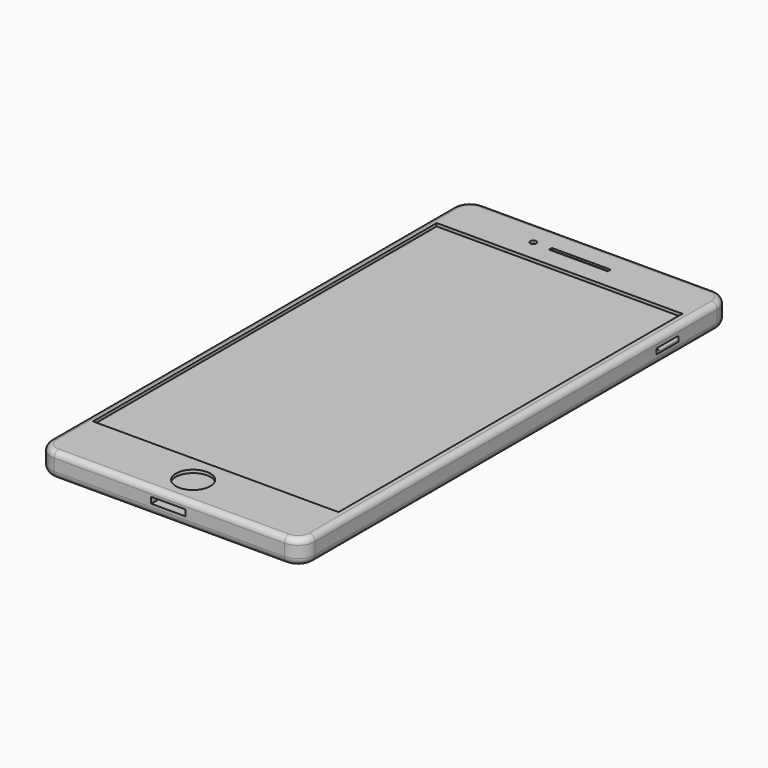
from build123d import *

# Parameters (mm, degrees)
F0_W         = 77.9
F0_H         = 158.2
F1_DEPTH     = 7.3
F2_R         = 5
F3_R         = 1.6899494937
F4_R         = 2.1727922061
F5_W         = 72.4303945899
F5_H         = 126.6588754952
F6_DEPTH     = 0.9
F7_R         = 5.0823894813
F8_DEPTH     = 0.9
F9_W         = 17.3039510846
F9_H         = 1.0814964771
F10_DEPTH    = 0.6
F11_R        = 0.8966339166
F12_DEPTH    = 0.8
F13_W        = 17.3039520159
F13_H        = 4.6321238935
F14_DEPTH    = 1.7
F15_R        = 0.7242640687
F16_R        = 1.0910584654
F17_DEPTH    = 1.2
F18_R        = 1.1204591048
F18_R_2      = 0.2597799208
F19_DEPTH    = 0.5
F20_R        = 0.5652467708
F21_DEPTH    = 1.3
F22_R        = 1.5140930758
F23_DEPTH    = 0.6
F24_W        = 10.0857308134
F24_H        = 1.8002798315
F25_DEPTH    = 8.7
F26_W        = 7.992297411
F26_H        = 1.5090261586
F27_DEPTH    = 0.5
F28_T1_DEPTH = 5.0389206483
F28_T3_DEPTH = 11.5221919007
F29_R        = 1.0914541248
F30_DEPTH    = 0.9
F31_R        = 1.1331057204
F32_DEPTH    = 0.8
F33_W        = 73.5544155877
F33_H        = 1.0814964771
F34_DEPTH    = 0.4


# Not quite as in the source:
# - a fillet or chamfer that OpenCascade refuses, or shapes differently, is made with other operations: its cross-section is extruded or revolved along the edge and cut away or added


with BuildPart() as f1:
    # F0 (on Top) → F1 (new body)
    with BuildSketch(Plane.XY):
        with Locations((-9.3765874773, -13.58352229)):
            Rectangle(F0_W, F0_H)
    extrude(amount=F1_DEPTH)

    # F2
    f2_edges = [f1.edges().sort_by_distance(p)[0] for p in [
        (-48.326587, -92.683522, 3.65),
        (29.573413, -92.683522, 3.65),
        (29.573413, 65.516478, 3.65),
        (-48.326587, 65.516478, 3.65),
    ]]
    fillet(f2_edges, radius=F2_R)

    # F3
    f3_edges = [f1.edges().sort_by_distance(p)[0] for p in [
        (-48.326587, -13.583522, 7.3),
        (-9.376587, 65.516478, 7.3),
        (28.108946, 64.052012, 7.3),
        (-46.862121, 64.052012, 7.3),
        (29.573413, -13.583522, 7.3),
        (28.108946, -91.219056, 7.3),
        (-46.862121, -91.219056, 7.3),
        (-9.376587, -92.683522, 7.3),
    ]]
    fillet(f3_edges, radius=F3_R)

    # F4
    f4_edges = [f1.edges().sort_by_distance(p)[0] for p in [
        (-48.326587, -13.583522, 0),
        (-9.376587, 65.516478, 0),
        (28.108946, 64.052012, 0),
        (-46.862121, 64.052012, 0),
        (29.573413, -13.583522, 0),
        (28.108946, -91.219056, 0),
        (-46.862121, -91.219056, 0),
        (-9.376587, -92.683522, 0),
    ]]
    fillet(f4_edges, radius=F4_R)

    # F5 (on face) → F6 (cut)
    with BuildSketch(Plane.XY.offset(7.3)):
        with Locations((-9.5828361809, -11.9932051748)):
            Rectangle(F5_W, F5_H)
    extrude(amount=-F6_DEPTH, mode=Mode.SUBTRACT)

    # F7 (on face) → F8 (cut)
    with BuildSketch(Plane.XY.offset(7.3)):
        with Locations((-9.5828361809, -83.671361208)):
            Circle(F7_R)
    extrude(amount=-F8_DEPTH, mode=Mode.SUBTRACT)

    # F9 (on face) → F10 (cut)
    with BuildSketch(Plane.XY.offset(7.3)):
        with Locations((-8.6519755423, 57.6703026891)):
            Rectangle(F9_W, F9_H)
    extrude(amount=-F10_DEPTH, mode=Mode.SUBTRACT)

    # F11 (on face) → F12 (cut)
    with BuildSketch(Plane.XY.offset(7.3)):
        with Locations((-22.4402733147, 57.7334612608)):
            Circle(F11_R)
    extrude(amount=-F12_DEPTH, mode=Mode.SUBTRACT)

    # F13 (on face) → F14 (join)
    with BuildSketch(Plane(origin=(0, 0, 0), x_dir=(1, 0, 0), z_dir=(0, 0, -1))):
        with Locations((11.9729838334, -58.2004157633)):
            Rectangle(F13_W, F13_H)
    extrude(amount=F14_DEPTH)

    # F15
    f15_edges = [f1.edges().sort_by_distance(p)[0] for p in [
        (11.972984, 60.516478, -1.7),
        (11.972984, 55.884354, -1.7),
        (20.62496, 58.200416, -1.7),
        (3.321008, 58.200416, -1.7),
    ]]
    fillet(f15_edges, radius=F15_R)

    # F16 (on face) → F17 (cut)
    with BuildSketch(Plane(origin=(0, 0, -1.7), x_dir=(1, 0, 0), z_dir=(0, 0, -1))):
        with Locations((17.652342096, -58.0027028918)):
            Circle(F16_R)
    extrude(amount=-F17_DEPTH, mode=Mode.SUBTRACT)

    # F18 (on face) → F19 (cut)
    with BuildSketch(Plane(origin=(0, 0, -1.7), x_dir=(1, 0, 0), z_dir=(0, 0, -1))):
        with Locations((13.1328506395, -57.9593703151)):
            Circle(F18_R)
        with Locations((13.1328506395, -57.9593703151)):
            Circle(F18_R_2, mode=Mode.SUBTRACT)
    extrude(amount=-F19_DEPTH, mode=Mode.SUBTRACT)

    # F20 (on face) → F21 (cut)
    with BuildSketch(Plane(origin=(0, 0, 0), x_dir=(1, 0, 0), z_dir=(0, 0, -1))):
        with Locations((0, -57.881783694)):
            Circle(F20_R)
    extrude(amount=-F21_DEPTH, mode=Mode.SUBTRACT)

    # F22 (on face) → F23 (cut)
    with BuildSketch(Plane(origin=(0, 0, 0), x_dir=(1, 0, 0), z_dir=(0, 0, -1))):
        with Locations((-3.8621318527, -57.8266605735)):
            Circle(F22_R)
    extrude(amount=-F23_DEPTH, mode=Mode.SUBTRACT)

    # F24 (on face) → F25 (cut)
    with BuildSketch(Plane.XZ.offset(92.68352229)):
        with Locations((-9.6801561303, 3.9914349327)):
            Rectangle(F24_W, F24_H)
    extrude(amount=-F25_DEPTH, mode=Mode.SUBTRACT)

    # F26 (on face) → F27 (join)
    with BuildSketch(Plane.YZ.offset(29.5734125227)):
        with Locations((42.0706942677, 3.8539019879)):
            Rectangle(F26_W, F26_H)
    extrude(amount=F27_DEPTH)

    # F28: fillet of radius 0.7484062043 on 4 edges, made by hand

    # F28_s2 → F28_t1 (cut)
    with BuildSketch(Plane.XY.offset(1.3344416637)):
        with BuildLine():
            ThreePointArc((29.5734125227, 46.0668429732), (29.9357520066, 45.7934164433), (30.0734125227, 45.3608640753))
            Line((30.0734125227, 45.3608640753), (30.0734125227, 46.0668429732))
            Line((30.0734125227, 46.0668429732), (29.5734125227, 46.0668429732))
        make_face()
        with BuildLine():
            ThreePointArc((29.5734125227, 38.0745455623), (29.9357520066, 38.3479720922), (30.0734125227, 38.7805244602))
            Line((30.0734125227, 38.7805244602), (30.0734125227, 38.0745455623))
            Line((30.0734125227, 38.0745455623), (29.5734125227, 38.0745455623))
        make_face()
    extrude(amount=F28_T1_DEPTH, mode=Mode.SUBTRACT)

    # F28_s4 → F28_t3 (cut)
    with BuildSketch(Plane.XZ.offset(-47.8317902181)):
        with BuildLine():
            ThreePointArc((29.5734125227, 4.6084150672), (29.9357520066, 4.3349885373), (30.0734125227, 3.9024361693))
            Line((30.0734125227, 3.9024361693), (30.0734125227, 4.6084150672))
            Line((30.0734125227, 4.6084150672), (29.5734125227, 4.6084150672))
        make_face()
        with BuildLine():
            ThreePointArc((29.5734125227, 3.0993889086), (29.9357520066, 3.3728154385), (30.0734125227, 3.8053678065))
            Line((30.0734125227, 3.8053678065), (30.0734125227, 3.0993889086))
            Line((30.0734125227, 3.0993889086), (29.5734125227, 3.0993889086))
        make_face()
    extrude(amount=F28_T3_DEPTH, mode=Mode.SUBTRACT)

    # F29 (on face) → F30 (join)
    with BuildSketch(Plane(origin=(-48.3265874773, 0, 0), x_dir=(0, -1, 0), z_dir=(-1, 0, 0))):
        with Locations((-41.7392961681, 4.070978146)):
            Circle(F29_R)
    extrude(amount=F30_DEPTH)

    # F31 (on face) → F32 (join)
    with BuildSketch(Plane(origin=(-48.3265874773, 0, 0), x_dir=(0, -1, 0), z_dir=(-1, 0, 0))):
        with Locations((-36.7904044688, 4.1209622286)):
            Circle(F31_R)
    extrude(amount=F32_DEPTH)

    # F33 (on face) → F34 (cut)
    with BuildSketch(Plane(origin=(0, 0, 0), x_dir=(1, 0, 0), z_dir=(0, 0, -1))):
        with Locations((-9.3765874773, 75.3538236022)):
            Rectangle(F33_W, F33_H)
    extrude(amount=-F34_DEPTH, mode=Mode.SUBTRACT)


solid = f1.part
